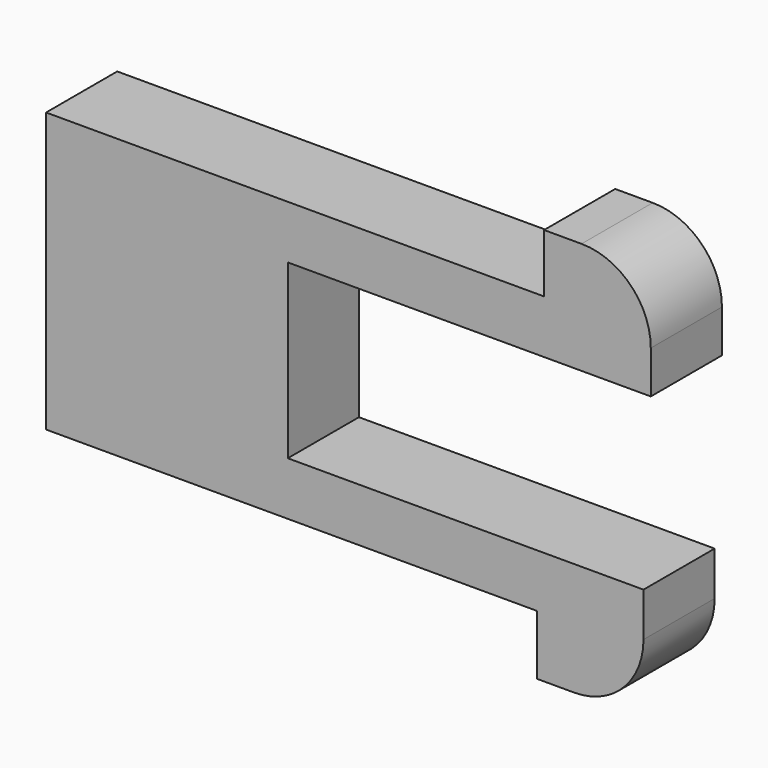
from build123d import *

# Parameters (mm, degrees)
F1_DEPTH = 2.5


# Not quite as in the source:
# - a feature names something its author has since deleted; it is built from what else it names


with BuildPart() as f1:
    # F0 (on Front) → F1 (new body)
    with BuildSketch(Plane.XZ):
        with BuildLine():
            Line((-16.7953648853, -9.0339062735), (-6.5833406376, -9.0339062735))
            Line((-6.5833406376, -9.0339062735), (-3, -9.0339062735))
            Line((-3, -9.0339062735), (-3, -10.7153228952))
            Line((-3, -10.7153228952), (-1.9461073071, -10.7153228952))
            ThreePointArc((-1.9461073071, -10.7153228952), (-0.5700016333, -10.1453212619), (0, -8.7692155881))
            Line((0, -8.7692155881), (0, -8.5))
            Line((0, -8.5), (0, -7.5339062735))
            Line((0, -7.5339062735), (-10, -7.5339062735))
            Line((-10, -7.5339062735), (-10, -2.6866213954))
            Line((-10, -2.6866213954), (0.2046351147, -2.6866213954))
            Line((0.2046351147, -2.6866213954), (0.2046351147, -1.7576624442))
            Line((0.2046351147, -1.7576624442), (0.2046351147, -1.4884468561))
            ThreePointArc((0.2046351147, -1.4884468561), (-0.3653665186, -0.1123411824), (-1.7414721924, 0.457660451))
            Line((-1.7414721924, 0.457660451), (-2.7953648853, 0.457660451))
            Line((-2.7953648853, 0.457660451), (-2.7953648853, -1.1866213954))
            Line((-2.7953648853, -1.1866213954), (-6.7360828114, -1.1866213954))
            Line((-6.7360828114, -1.1866213954), (-16.7953648853, -1.1866213954))
            Line((-16.7953648853, -1.1866213954), (-16.7953648853, -9.0339062735))
        make_face()
    extrude(amount=F1_DEPTH)


solid = f1.part
